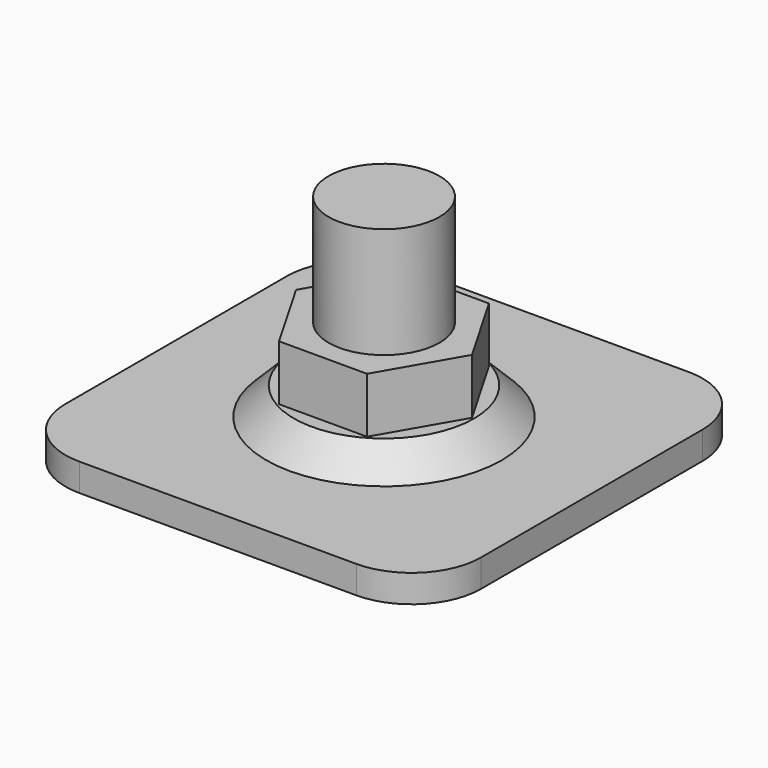
from build123d import *

# Parameters (mm, degrees)
F1_DEPTH = 2
F2_R     = 8.5
F3_DEPTH = 2
F4_SIZE  = 1.99999
F6_DEPTH = 4
F7_R     = 4
F8_DEPTH = 8


# Not quite as in the source:
# - a fillet or chamfer is up to 0.001 mm smaller than in the source, because OpenCascade refuses the exact size


with BuildPart() as f1:
    # F0 (on Top) → F1 (new body)
    with BuildSketch(Plane.XY):
        with BuildLine():
            ThreePointArc((15, 10), (13.5355339059, 13.5355339059), (10, 15))
            Line((10, 15), (-10, 15))
            ThreePointArc((-10, 15), (-13.5355339059, 13.5355339059), (-15, 10))
            Line((-15, 10), (-15, -10))
            ThreePointArc((-15, -10), (-13.5355339059, -13.5355339059), (-10, -15))
            Line((-10, -15), (10, -15))
            ThreePointArc((10, -15), (13.5355339059, -13.5355339059), (15, -10))
            Line((15, -10), (15, 10))
        make_face()
    extrude(amount=F1_DEPTH)

    # F2 (on face) → F3 (join)
    with BuildSketch(Plane.XY.offset(2)):
        Circle(F2_R)
    extrude(amount=F3_DEPTH)

    # F4 (size 2 in the source; OpenCascade refuses exactly that, so slightly less here)
    f4_edges = [f1.edges().sort_by_distance(p)[0] for p in [
        (-8.5, 0, 4),
    ]]
    chamfer(f4_edges, length=F4_SIZE)

    # F5 (on face) → F6 (join)
    with BuildSketch(Plane.XY.offset(4)):
        Polygon((6.3508529611, 0), (3.1754264805, 5.5), (-3.1754264805, 5.5), (-6.3508529611, 0), (-3.1754264805, -5.5), (3.1754264805, -5.5), align=None)
    extrude(amount=F6_DEPTH)

    # F7 (on face) → F8 (join)
    with BuildSketch(Plane.XY.offset(8)):
        Circle(F7_R)
    extrude(amount=F8_DEPTH)


solid = f1.part
